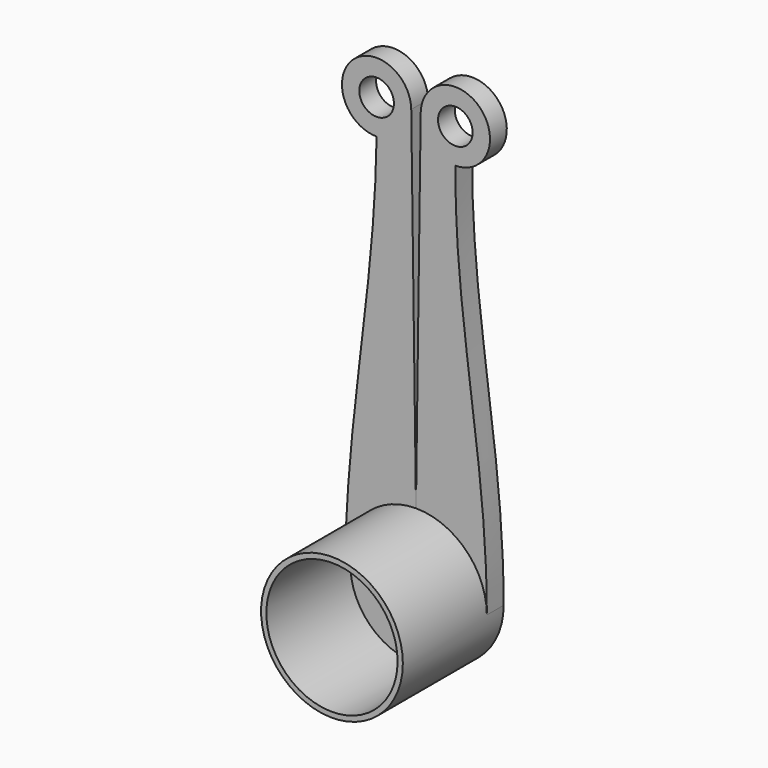
from build123d import *

# Parameters (mm, degrees)
F0_R     = 17.145
F0_R_2   = 15.875
F1_DEPTH = 25.4
F2_R     = 17.145
F3_DEPTH = 5.08
F4_R     = 4.191
F5_DEPTH = 5.08


# Not quite as in the source:
# - after a boolean that leaves OpenCascade's solid faulty, fix() repairs it


with BuildPart() as f1:
    # F0 (on Front) → F1 (new body)
    with BuildSketch(Plane.XZ):
        Circle(F0_R)
        Circle(F0_R_2, mode=Mode.SUBTRACT)
    extrude(amount=F1_DEPTH)

    # F2 (on face) → F3 (join)
    with BuildSketch(Plane(origin=(0, 0, 0), x_dir=(-1, 0, 0), z_dir=(0, 1, 0))):
        Circle(F2_R)
    extrude(amount=F3_DEPTH)

    # F4 (on face) → F5 (join, through all)
    with BuildSketch(Plane.XZ):
        with BuildLine():
            add(Edge.make_bspline(
                [(9.525, 93.218), (9.3322422676, 59.4415284404), (17.145, 33.7770215762), (17.145, 0)],
                knots=[0, 0, 0, 0, 93.5289256006, 93.5289256006, 93.5289256006, 93.5289256006], degree=3))
            ThreePointArc((9.525, 93.218), (15.4919111989, 107.486755876), (1.1437665087, 101.7133541532))
            Line((1.1437665087, 101.7133541532), (0, 17.145))
            ThreePointArc((0, 17.145), (12.1233457634, 12.1233457634), (17.145, 0))
        make_face()
        with Locations((9.525, 101.6)):
            Circle(F4_R, mode=Mode.SUBTRACT)
        with BuildLine():
            ThreePointArc((-17.1425003406, 0.2927577006), (-12.0193946233, 12.2264131244), (0, 17.145))
            Line((0, 17.145), (-1.1437665087, 101.7133541532))
            ThreePointArc((-1.1437665087, 101.7133541532), (-15.4919111989, 107.486755876), (-9.525, 93.218))
            add(Edge.make_bspline(
                [(-9.525, 93.218), (-10.0234570054, 59.5641158888), (-16.5685631435, 33.8997937459), (-17.1425003406, 0.2927577006)],
                knots=[0, 0, 0, 0, 93.2585047549, 93.2585047549, 93.2585047549, 93.2585047549], degree=3))
        make_face()
        with Locations((-9.525, 101.6)):
            Circle(F4_R, mode=Mode.SUBTRACT)
    extrude(amount=-F5_DEPTH)

    add(f1.part.fix(), mode=Mode.REPLACE)


solid = f1.part
